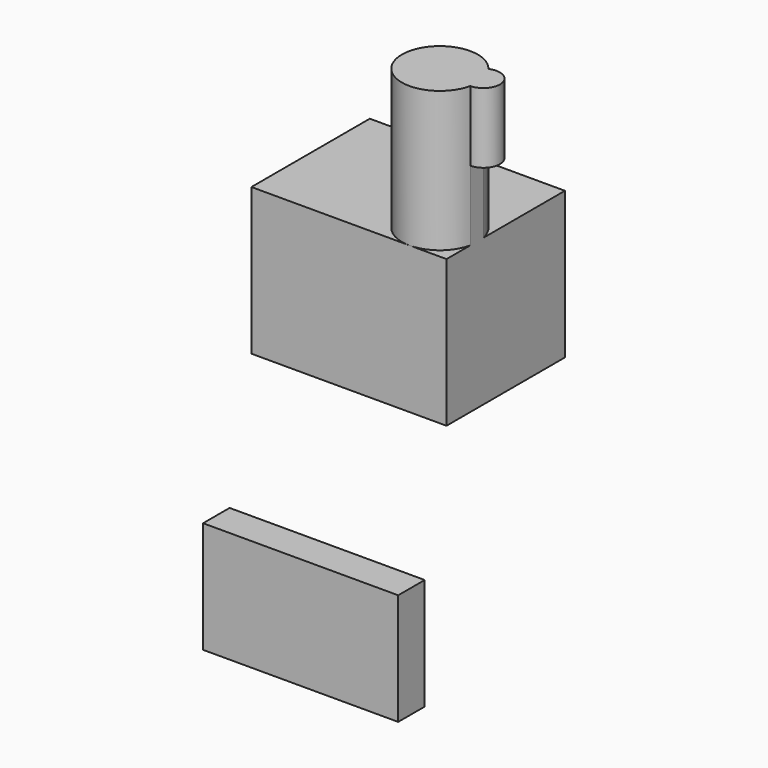
from build123d import *

# Parameters (mm, degrees)
F3_W     = 12.0016336441
F3_H     = 40.3636842966
F0_DEPTH = 70.6501286477
F3_W_2   = 53.5843074322
F3_H_2   = 53.1327724457
F4_DEPTH = 25.4
F2_R     = 5.9481463901
F5_DEPTH = 25.4


with BuildPart() as f0:
    # F3 (on Right) → F0 (new body)
    with BuildSketch(Plane.YZ):
        with Locations((-47.5331246853, -50.7349595428)):
            Rectangle(F3_W, F3_H)
    extrude(amount=F0_DEPTH)


with BuildPart() as f0b:
    # F3 (on Right) → F0, piece 2 (new body)
    with BuildSketch(Plane.YZ):
        with Locations((-4.8692375422, 41.1562174559)):
            Rectangle(F3_W_2, F3_H_2)
    extrude(amount=F0_DEPTH)

    # F1 (on face) → F4 (join)
    with BuildSketch(Plane.XY.offset(67.7226036787)):
        with BuildLine():
            Line((70.6501286477, -20.8966161843), (70.6501286477, -14.9484697942))
            ThreePointArc((70.6501286477, -14.9484697942), (46.5221876519, -9.3232519897), (57.2370439768, -31.6613912582))
            ThreePointArc((57.2370439768, -31.6613912582), (65.8363349764, -28.6373993141), (70.6501286477, -20.8966161843))
        make_face()
    extrude(amount=F4_DEPTH)

    # F2 (on face) → F5 (join)
    with BuildSketch(Plane.XY.offset(93.1226036787)):
        with Locations((70.6501286477, -14.9484697942)):
            Circle(F2_R)
        with BuildLine():
            ThreePointArc((57.2370439768, -31.6613912582), (65.8363349764, -28.6373993141), (70.6501286477, -20.8966161843))
            ThreePointArc((70.6501286477, -20.8966161843), (64.8430195216, -16.2360757414), (68.1359779337, -9.5577841546))
            ThreePointArc((68.1359779337, -9.5577841546), (44.914744999, -11.8466151045), (57.2370439768, -31.6613912582))
        make_face()
    extrude(amount=F5_DEPTH)


solid = Compound([f0.part, f0b.part])
